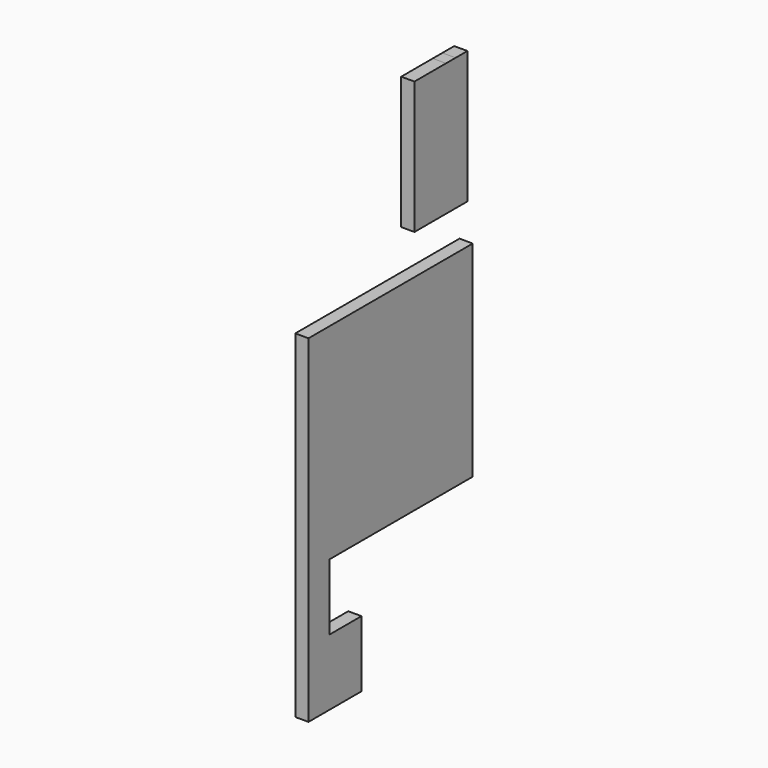
from build123d import *

# Parameters (mm, degrees)
F0_W     = 0.25
F0_H     = 15
F1_DEPTH = 1


# Not quite as in the source:
# - a feature names something its author has since deleted; it is built from what else it names


with BuildPart() as f1:
    # F0 (on Right) → F1 (new body)
    with BuildSketch(Plane.YZ):
        Polygon((11.5, 0), (0, 0), (-1.75, 0), (-1.75, -15), (0, -15), (4.35, -15), (7.15, -15), (11.5, -15), (13.25, -15), (13.25, 0), align=None)
        with Locations((-1.875, -7.5)):
            Rectangle(F0_W, F0_H)
        with Locations((13.375, -7.5)):
            Rectangle(F0_W, F0_H)
        Polygon((0, -15), (-1.75, -15), (-2, -15), (-2, -15.5), (0, -15.5), (13.5, -15.5), (13.5, -15), (13.25, -15), (11.5, -15), (7.15, -15), (4.35, -15), align=None)
        Polygon((0, -15.5), (-2, -15.5), (-2, -25.5), (3, -25.5), (3, -20.5), (0, -20.5), align=None)
    extrude(amount=F1_DEPTH)


with BuildPart() as f1b:
    # F0 (on Right) → F1, piece 2 (new body)
    with BuildSketch(Plane.YZ):
        Polygon((10.9789912227, 13.000000208), (8.0000062163, 13.0000000082), (8.0000066322, 2.9999998385), (10.9789916386, 2.9999997318), (11.3841416386, 2.9999997318), (11.8841416386, 2.9999997318), (13.0000016386, 2.9999997782), (13.0000012227, 13.0000002544), (11.8841412227, 13.000000208), (11.3841412227, 13.000000208), align=None)
    extrude(amount=F1_DEPTH)


solid = Compound([f1.part, f1b.part])
